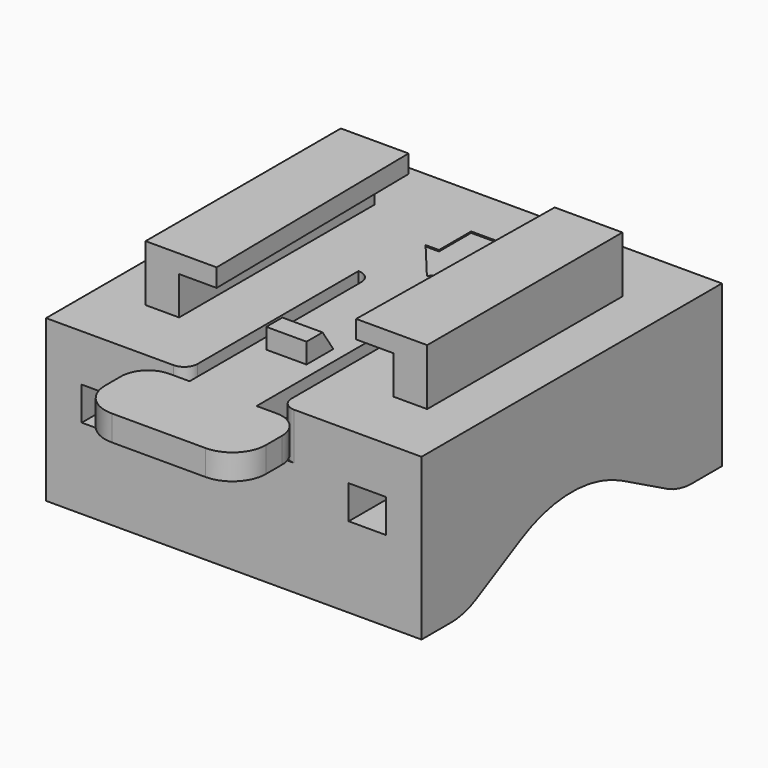
from build123d import *

# Parameters (mm, degrees)
F1_DEPTH  = 14
F3_W      = 7
F3_H      = 3.5
F4_DEPTH  = 16
F5_W      = 5
F5_H      = 0.4111507442
F5_H_2    = 17
F6_DEPTH  = 1.9
F8_R      = 0.99999
F10_DEPTH = 1.5
F11_W     = 2.5
F11_H     = 18.2
F12_DEPTH = 4.2
F13_W     = 2.5
F13_H     = 18.2
F14_DEPTH = 1.35
F15_W     = 3
F15_H     = 3
F16_DEPTH = 0.1
F17_DEPTH = 15
F18_R     = 5
F19_W     = 2.0917450339
F19_H     = 2.5
F20_DEPTH = 28.001
F19_W_2   = 2.772427164
F21_DEPTH = 28.001


# Not quite as in the source:
# - a fillet or chamfer is up to 0.001 mm smaller than in the source, because OpenCascade refuses the exact size
# - the program builds the solid bodies; features that only make, move or delete a surface that nothing else refers to are left out


with BuildPart() as f1:
    # F0 (on Front) → F1 (new body, symmetric)
    with BuildSketch(Plane.XZ):
        with BuildLine():
            Line((10, -6), (14, -6))
            Line((14, -6), (14, 6))
            Line((14, 6), (-14, 6))
            Line((-14, 6), (-14, -6))
            Line((-14, -6), (-10, -6))
            Line((-10, -6), (-4.7058823529, -3.1764705882))
            ThreePointArc((-4.7058823529, -3.1764705882), (0, -2), (4.7058823529, -3.1764705882))
            Line((4.7058823529, -3.1764705882), (10, -6))
        make_face()
        with BuildLine():
            Line((-10, -6), (10, -6))
            Line((10, -6), (4.7058823529, -3.1764705882))
            ThreePointArc((4.7058823529, -3.1764705882), (0, -2), (-4.7058823529, -3.1764705882))
            Line((-4.7058823529, -3.1764705882), (-10, -6))
        make_face()
    extrude(amount=F1_DEPTH, both=True)

    # F3 (on face) → F4 (cut)
    with BuildSketch(Plane.XZ.offset(14)):
        with Locations((0, 4.25)):
            Rectangle(F3_W, F3_H)
    extrude(amount=-F4_DEPTH, mode=Mode.SUBTRACT)

    # F5 (on face) → F6 (join)
    with BuildSketch(Plane.XY.offset(6)):
        with BuildLine():
            Line((2.5, -15), (-2.5, -15))
            Line((-2.5, -15), (-4, -15))
            ThreePointArc((-4, -15), (-5.4142135624, -15.5857864376), (-6, -17))
            Line((-6, -17), (-6, -18.5))
            ThreePointArc((-6, -18.5), (-5.267766953, -20.267766953), (-3.5, -21))
            Line((-3.5, -21), (3.5, -21))
            ThreePointArc((3.5, -21), (5.267766953, -20.267766953), (6, -18.5))
            Line((6, -18.5), (6, -17))
            ThreePointArc((6, -17), (5.4142135624, -15.5857864376), (4, -15))
            Line((4, -15), (2.5, -15))
        make_face()
        with Locations((0, 2.2055753721)):
            Rectangle(F5_W, F5_H)
        with Locations((0, -6.5)):
            Rectangle(F5_W, F5_H_2)
    extrude(amount=-F6_DEPTH)

    # F7: union 

    # F8 (radius 1 in the source; OpenCascade refuses exactly that, so slightly less here)
    f8_edges = [f1.edges().sort_by_distance(p)[0] for p in [
        (-3.5, -14, 4.25),
        (3.5, -14, 4.25),
        (2.5, 2, 5.05),
        (-2.5, 2, 5.05),
    ]]
    fillet(f8_edges, radius=F8_R)

    # F9 (on Right) → F10 (join, symmetric)
    with BuildSketch(Plane.YZ):
        Polygon((-6.6, 6), (-7.6, 7.5), (-9.1, 7.5), (-9.1, 6), align=None)
    extrude(amount=F10_DEPTH, both=True)

    # F11 (on face) → F12 (join)
    with BuildSketch(Plane.XY.offset(6)):
        with Locations((-9.25, 0)):
            Rectangle(F11_W, F11_H)
        with Locations((9.25, 0)):
            Rectangle(F11_W, F11_H)
    extrude(amount=F12_DEPTH)

    # F13 (on face) → F14 (join)
    with BuildSketch(Plane.XY.offset(10.2)):
        with Locations((-9.25, 0)):
            Rectangle(F13_W, F13_H)
        Polygon((-5.45, 9.1), (-8, 9.1), (-8, -9.1), (-5.2, -9.1), align=None)
        Polygon((5.45, 9.1), (5.2, -9.1), (10.5, -9.1), (10.5, 9.1), align=None)
    extrude(amount=-F14_DEPTH)

    # F15 (on face) → F16 (cut)
    with BuildSketch(Plane.XY.offset(6)):
        with Locations((0, 8.5)):
            Rectangle(F15_W, F15_H)
        Polygon((2.5, 7), (1.5, 7), (-1.5, 7), (-2.5, 7), (0, 4), align=None)
    extrude(amount=-F16_DEPTH, mode=Mode.SUBTRACT)

    # F2 (on Right) → F17 (cut, symmetric)
    with BuildSketch(Plane.YZ):
        with BuildLine():
            Line((-10, -6), (10, -6))
            Line((10, -6), (4.7058823529, -3.1764705882))
            ThreePointArc((4.7058823529, -3.1764705882), (0, -2), (-4.7058823529, -3.1764705882))
            Line((-4.7058823529, -3.1764705882), (-10, -6))
        make_face()
    extrude(amount=F17_DEPTH, both=True, mode=Mode.SUBTRACT)

    # F18
    f18_edges = [f1.edges().sort_by_distance(p)[0] for p in [
        (0, -10, -6),
        (0, 10, -6),
    ]]
    fillet(f18_edges, radius=F18_R)

    # F19 (on face) → F20 (cut, through all)
    with BuildSketch(Plane.XZ.offset(14)):
        with Locations((-10.2958725169, 1.25)):
            Rectangle(F19_W, F19_H)
    extrude(amount=-F20_DEPTH, mode=Mode.SUBTRACT)

    # F19 (on face) → F21 (cut, through all)
    with BuildSketch(Plane.XZ.offset(14)):
        with Locations((-10.2958725169, 1.25)):
            Rectangle(F19_W, F19_H)
        with Locations((9.9555305205, 1.25)):
            Rectangle(F19_W_2, F19_H)
    extrude(amount=-F21_DEPTH, mode=Mode.SUBTRACT)


solid = f1.part
